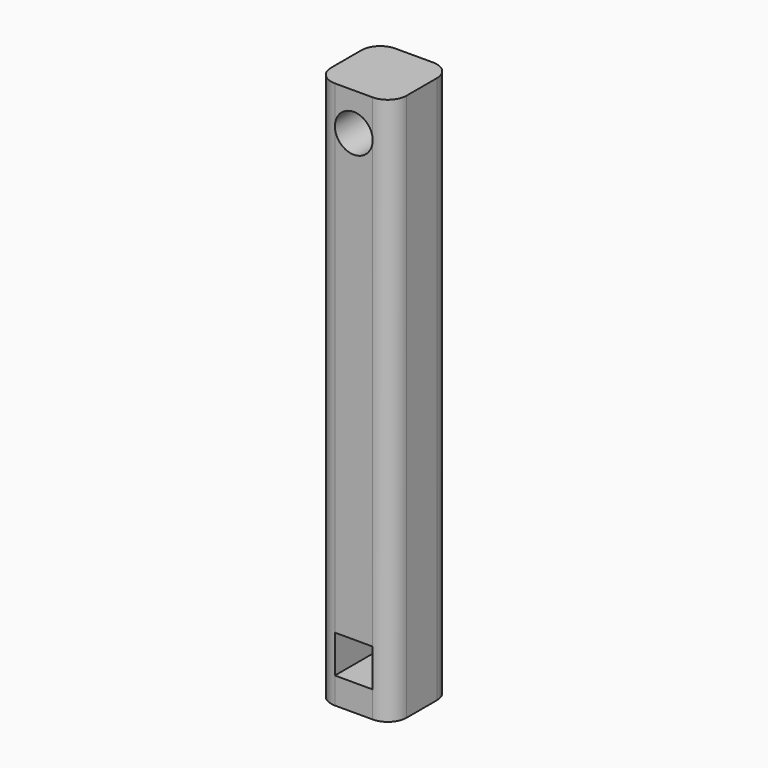
from build123d import *

# Parameters (mm, degrees)
F1_DEPTH = 25.4
F3_D     = 12.7
F3_DEPTH = 254
F3_TIP   = 3.8154649308
F4_W     = 25.4
F4_H     = 82.55
F5_DEPTH = 25.4
F7_DEPTH = 25.4
F8_R     = 6.34999


# Not quite as in the source:
# - a fillet or chamfer is up to 0.001 mm smaller than in the source, because OpenCascade refuses the exact size


with BuildPart() as f1:
    # F0 (on Front) → F1 (new body)
    with BuildSketch(Plane.XZ):
        Polygon((-12.7, -32.0098340811), (0, -32.0098340811), (12.7, -32.0098340811), (12.7, 69.5901659189), (-12.7, 69.5901659189), align=None)
    extrude(amount=F1_DEPTH)

    # F3
    with Locations(Plane.XZ.offset(25.4)):
        with Locations((0, 56.8901659189)):
            Hole(F3_D / 2, depth=F3_DEPTH)
            with Locations((0, 0, -(F3_DEPTH + F3_TIP / 2))):  # 118° drill point
                Cone(0, F3_D / 2, F3_TIP, mode=Mode.SUBTRACT)

    # F4 (on face) → F5 (join)
    with BuildSketch(Plane.XZ.offset(25.4)):
        with Locations((0, -73.2848340811)):
            Rectangle(F4_W, F4_H)
    extrude(amount=-F5_DEPTH)

    # F6 (on face) → F7 (cut)
    with BuildSketch(Plane(origin=(0, 0, 0), x_dir=(-1, 0, 0), z_dir=(0, 1, 0))):
        Polygon((0, -105.6698340811), (6.35, -105.6698340811), (6.35, -92.9698340811), (-6.35, -92.9698340811), (-6.35, -105.6698340811), align=None)
    extrude(amount=-F7_DEPTH, mode=Mode.SUBTRACT)

    # F8 (radius 6.35 in the source; OpenCascade refuses exactly that, so slightly less here)
    f8_edges = [f1.edges().sort_by_distance(p)[0] for p in [
        (12.7, 0, -22.484834),
        (-12.7, 0, -22.484834),
        (-12.7, -25.4, -22.484834),
        (12.7, -25.4, -22.484834),
    ]]
    fillet(f8_edges, radius=F8_R)


solid = f1.part
